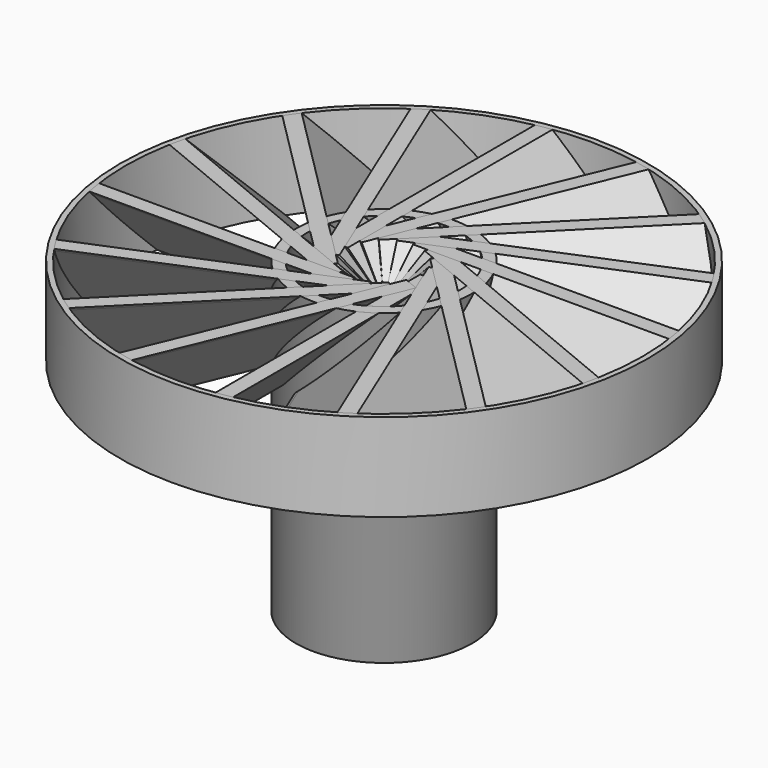
from build123d import *

# Parameters (mm, degrees)
F0_R     = 25.4
F0_R_2   = 22.225
F1_DEPTH = 88.9
F2_R     = 76.2
F2_R_2   = 74.6125
F3_DEPTH = 25.4
F5_REACH = 115.4257339758
F6_COUNT = 16


with BuildPart() as f1:
    # F0 (on Top) → F1 (new body)
    with BuildSketch(Plane.XY):
        Circle(F0_R)
        Circle(F0_R_2, mode=Mode.SUBTRACT)
    extrude(amount=-F1_DEPTH)


with BuildPart() as f3:
    # F2 (on Top) → F3 (new body)
    with BuildSketch(Plane.XY):
        Circle(F2_R)
        Circle(F2_R_2, mode=Mode.SUBTRACT)
    extrude(amount=-F3_DEPTH)


with BuildPart() as f5:
    f5_end = f3.part.faces().sort_by_distance((-74.6125, 0, -12.7))[0]
    # F4 (on Front) → F5 (new body, up to a face of F3 that its end follows)
    with BuildSketch(Plane.XZ):
        Polygon((-13.8225320151, -24.2774679849), (-14.9450640303, -25.4), (-10.4549359697, -25.4), (13.8225320151, -1.1225320151), (14.9450640303, 0), (10.4549359697, 0), align=None)
    f5_long = extrude(amount=F5_REACH, mode=Mode.PRIVATE)
    add(split(f5_long, bisect_by=f5_end, keep=Keep.TOP, mode=Mode.PRIVATE))


with BuildPart() as f6_1:
    # F6: instance of F1
    add(f1.part.rotate(Axis((0, 0, 0), (0, 0, 1)), 1 * 360 / F6_COUNT))


with BuildPart() as f6_2:
    # F6: instance of F1
    add(f1.part.rotate(Axis((0, 0, 0), (0, 0, 1)), 2 * 360 / F6_COUNT))


with BuildPart() as f6_3:
    # F6: instance of F1
    add(f1.part.rotate(Axis((0, 0, 0), (0, 0, 1)), 3 * 360 / F6_COUNT))


with BuildPart() as f6_4:
    # F6: instance of F1
    add(f1.part.rotate(Axis((0, 0, 0), (0, 0, 1)), 4 * 360 / F6_COUNT))


with BuildPart() as f6_5:
    # F6: instance of F1
    add(f1.part.rotate(Axis((0, 0, 0), (0, 0, 1)), 5 * 360 / F6_COUNT))


with BuildPart() as f6_6:
    # F6: instance of F1
    add(f1.part.rotate(Axis((0, 0, 0), (0, 0, 1)), 6 * 360 / F6_COUNT))


with BuildPart() as f6_7:
    # F6: instance of F1
    add(f1.part.rotate(Axis((0, 0, 0), (0, 0, 1)), 7 * 360 / F6_COUNT))


with BuildPart() as f6_8:
    # F6: instance of F1
    add(f1.part.rotate(Axis((0, 0, 0), (0, 0, 1)), 8 * 360 / F6_COUNT))


with BuildPart() as f6_9:
    # F6: instance of F1
    add(f1.part.rotate(Axis((0, 0, 0), (0, 0, 1)), 9 * 360 / F6_COUNT))


with BuildPart() as f6_10:
    # F6: instance of F1
    add(f1.part.rotate(Axis((0, 0, 0), (0, 0, 1)), 10 * 360 / F6_COUNT))


with BuildPart() as f6_11:
    # F6: instance of F1
    add(f1.part.rotate(Axis((0, 0, 0), (0, 0, 1)), 11 * 360 / F6_COUNT))


with BuildPart() as f6_12:
    # F6: instance of F1
    add(f1.part.rotate(Axis((0, 0, 0), (0, 0, 1)), 12 * 360 / F6_COUNT))


with BuildPart() as f6_13:
    # F6: instance of F1
    add(f1.part.rotate(Axis((0, 0, 0), (0, 0, 1)), 13 * 360 / F6_COUNT))


with BuildPart() as f6_14:
    # F6: instance of F1
    add(f1.part.rotate(Axis((0, 0, 0), (0, 0, 1)), 14 * 360 / F6_COUNT))


with BuildPart() as f6_15:
    # F6: instance of F1
    add(f1.part.rotate(Axis((0, 0, 0), (0, 0, 1)), 15 * 360 / F6_COUNT))


with BuildPart() as f6_16:
    # F6: instance of F5
    add(f5.part.rotate(Axis((0, 0, 0), (0, 0, 1)), 1 * 360 / F6_COUNT))


with BuildPart() as f6_17:
    # F6: instance of F5
    add(f5.part.rotate(Axis((0, 0, 0), (0, 0, 1)), 2 * 360 / F6_COUNT))


with BuildPart() as f6_18:
    # F6: instance of F5
    add(f5.part.rotate(Axis((0, 0, 0), (0, 0, 1)), 3 * 360 / F6_COUNT))


with BuildPart() as f6_19:
    # F6: instance of F5
    add(f5.part.rotate(Axis((0, 0, 0), (0, 0, 1)), 4 * 360 / F6_COUNT))


with BuildPart() as f6_20:
    # F6: instance of F5
    add(f5.part.rotate(Axis((0, 0, 0), (0, 0, 1)), 5 * 360 / F6_COUNT))


with BuildPart() as f6_21:
    # F6: instance of F5
    add(f5.part.rotate(Axis((0, 0, 0), (0, 0, 1)), 6 * 360 / F6_COUNT))


with BuildPart() as f6_22:
    # F6: instance of F5
    add(f5.part.rotate(Axis((0, 0, 0), (0, 0, 1)), 7 * 360 / F6_COUNT))


with BuildPart() as f6_23:
    # F6: instance of F5
    add(f5.part.rotate(Axis((0, 0, 0), (0, 0, 1)), 8 * 360 / F6_COUNT))


with BuildPart() as f6_24:
    # F6: instance of F5
    add(f5.part.rotate(Axis((0, 0, 0), (0, 0, 1)), 9 * 360 / F6_COUNT))


with BuildPart() as f6_25:
    # F6: instance of F5
    add(f5.part.rotate(Axis((0, 0, 0), (0, 0, 1)), 10 * 360 / F6_COUNT))


with BuildPart() as f6_26:
    # F6: instance of F5
    add(f5.part.rotate(Axis((0, 0, 0), (0, 0, 1)), 11 * 360 / F6_COUNT))


with BuildPart() as f6_27:
    # F6: instance of F5
    add(f5.part.rotate(Axis((0, 0, 0), (0, 0, 1)), 12 * 360 / F6_COUNT))


with BuildPart() as f6_28:
    # F6: instance of F5
    add(f5.part.rotate(Axis((0, 0, 0), (0, 0, 1)), 13 * 360 / F6_COUNT))


with BuildPart() as f6_29:
    # F6: instance of F5
    add(f5.part.rotate(Axis((0, 0, 0), (0, 0, 1)), 14 * 360 / F6_COUNT))


with BuildPart() as f6_30:
    # F6: instance of F5
    add(f5.part.rotate(Axis((0, 0, 0), (0, 0, 1)), 15 * 360 / F6_COUNT))


solid = Compound([f1.part, f3.part, f5.part, f6_1.part, f6_2.part, f6_3.part, f6_4.part, f6_5.part, f6_6.part, f6_7.part, f6_8.part, f6_9.part, f6_10.part, f6_11.part, f6_12.part, f6_13.part, f6_14.part, f6_15.part, f6_16.part, f6_17.part, f6_18.part, f6_19.part, f6_20.part, f6_21.part, f6_22.part, f6_23.part, f6_24.part, f6_25.part, f6_26.part, f6_27.part, f6_28.part, f6_29.part, f6_30.part])
